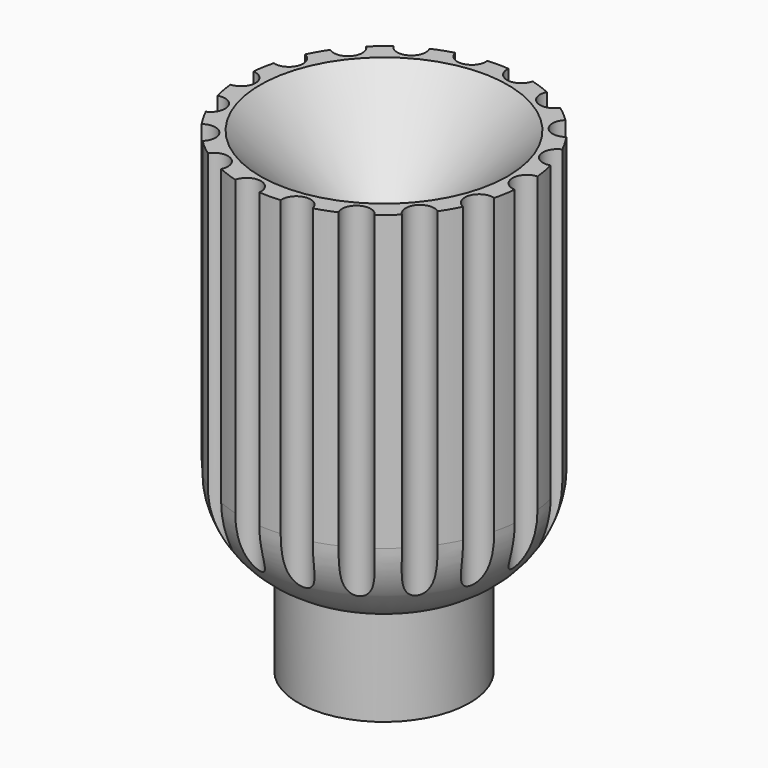
from build123d import *

# Parameters (mm, degrees)
F0_R     = 4.5
F0_R_2   = 1.5
F1_DEPTH = 5
F2_R     = 7.5
F2_R_2   = 1.5
F3_DEPTH = 20
F5_SIZE  = 5
F7_DEPTH = 25


# Not quite as in the source:
# - a fillet or chamfer that OpenCascade refuses, or shapes differently, is made with other operations: its cross-section is extruded or revolved along the edge and cut away or added


with BuildPart() as f1:
    # F0 (on Top) → F1 (new body)
    with BuildSketch(Plane.XY):
        Circle(F0_R)
        Circle(F0_R_2, mode=Mode.SUBTRACT)
    extrude(amount=F1_DEPTH)

    # F2 (on face) → F3 (join)
    with BuildSketch(Plane.XY.offset(5)):
        Circle(F2_R)
        Circle(F2_R_2, mode=Mode.SUBTRACT)
    extrude(amount=F3_DEPTH)

    # F4: fillet of radius 5 on 1 edges, made by hand

    # F4_s1 → F4_t2 (revolve, cut)
    with BuildSketch(Plane.XZ):
        with BuildLine():
            ThreePointArc((4.5, 5), (6.6833001327, 6.8439629074), (7.5, 9.582575695))
            Line((7.5, 9.582575695), (7.5, 5))
            Line((7.5, 5), (4.5, 5))
        make_face()
    revolve(axis=Axis((0, 0, 5), (0, 0, 1)), mode=Mode.SUBTRACT)

    # F5
    f5_edges = [f1.edges().sort_by_distance(p)[0] for p in [
        (-1.5, 0, 25),
    ]]
    chamfer(f5_edges, length=F5_SIZE)

    # F6 (on face) → F7 (cut)
    with BuildSketch(Plane.XY.offset(25)):
        with BuildLine():
            ThreePointArc((-7.4625, -0.7490619133), (-6.956573372, -0.5169018282), (-6.75, 0))
            ThreePointArc((-6.75, 0), (-6.956573372, 0.5169018282), (-7.4625, 0.7490619133))
            ThreePointArc((-7.4625, 0.7490619133), (-7.5, 0), (-7.4625, -0.7490619133))
        make_face()
        with BuildLine():
            ThreePointArc((-7.4625, -0.7490619133), (-7.5, 0), (-7.4625, 0.7490619133))
            ThreePointArc((-7.4625, 0.7490619133), (-8.25, 0), (-7.4625, -0.7490619133))
        make_face()
        with BuildLine():
            ThreePointArc((-6.7562619197, 3.256213272), (-7.0476946559, 2.5651510749), (-7.2686504456, 1.8484373671))
            ThreePointArc((-7.2686504456, 1.8484373671), (-6.60228296, 1.9617371033), (-6.2976946559, 2.5651510749))
            ThreePointArc((-6.2976946559, 2.5651510749), (-6.422764839, 2.9798349593), (-6.7562619197, 3.256213272))
        make_face()
        with BuildLine():
            ThreePointArc((-6.7562619197, -3.256213272), (-7.0476946559, -2.5651510749), (-7.2686504456, -1.8484373671))
            ThreePointArc((-7.2686504456, -1.8484373671), (-7.7524641215, -2.8216661824), (-6.7562619197, -3.256213272))
        make_face()
        with BuildLine():
            ThreePointArc((-6.2976946559, -2.5651510749), (-6.60228296, -1.9617371033), (-7.2686504456, -1.8484373671))
            ThreePointArc((-7.2686504456, -1.8484373671), (-7.0476946559, -2.5651510749), (-6.7562619197, -3.256213272))
            ThreePointArc((-6.7562619197, -3.256213272), (-6.422764839, -2.9798349593), (-6.2976946559, -2.5651510749))
        make_face()
        with BuildLine():
            ThreePointArc((-5.23511894, 5.3706172535), (-5.7453333234, 4.8209070726), (-6.1980943736, 4.222987821))
            ThreePointArc((-6.1980943736, 4.222987821), (-5.4114701685, 4.1493153858), (-4.9953333234, 4.8209070726))
            ThreePointArc((-4.9953333234, 4.8209070726), (-5.0578884938, 5.1207730531), (-5.23511894, 5.3706172535))
        make_face()
        with BuildLine():
            ThreePointArc((-4.9953333234, -4.8209070726), (-5.4114701685, -4.1493153858), (-6.1980943736, -4.222987821))
            ThreePointArc((-6.1980943736, -4.222987821), (-5.7453333234, -4.8209070726), (-5.23511894, -5.3706172535))
            ThreePointArc((-5.23511894, -5.3706172535), (-5.0578884938, -5.1207730531), (-4.9953333234, -4.8209070726))
        make_face()
        with BuildLine():
            ThreePointArc((-3.082543354, 6.8372455324), (-3.75, 6.4951905284), (-4.379956646, 6.0881836191))
            ThreePointArc((-4.379956646, 6.0881836191), (-3.5378296492, 5.7758270999), (-3, 6.4951905284))
            ThreePointArc((-3, 6.4951905284), (-3.020927821, 6.6711273289), (-3.082543354, 6.8372455324))
        make_face()
        with BuildLine():
            ThreePointArc((-3, -6.4951905284), (-3.5378296492, -5.7758270999), (-4.379956646, -6.0881836191))
            ThreePointArc((-4.379956646, -6.0881836191), (-3.75, -6.4951905284), (-3.082543354, -6.8372455324))
            ThreePointArc((-3.082543354, -6.8372455324), (-3.020927821, -6.6711273289), (-3, -6.4951905284))
        make_face()
        with BuildLine():
            ThreePointArc((-0.5581675461, 7.4792010931), (-1.3023613325, 7.3860581476), (-2.0335315056, 7.2190546206))
            ThreePointArc((-2.0335315056, 7.2190546206), (-1.2183304745, 6.6407804712), (-0.5523613325, 7.3860581476))
            ThreePointArc((-0.5523613325, 7.3860581476), (-0.5538142933, 7.4327200175), (-0.5581675461, 7.4792010931))
        make_face()
        with BuildLine():
            ThreePointArc((-0.5581675461, 7.4792010931), (-1.4325974658, 8.1246639624), (-2.0335315056, 7.2190546206))
            ThreePointArc((-2.0335315056, 7.2190546206), (-1.3023613325, 7.3860581476), (-0.5581675461, 7.4792010931))
        make_face()
        with BuildLine():
            ThreePointArc((-0.5523613325, -7.3860581476), (-1.2183304745, -6.6407804712), (-2.0335315056, -7.2190546206))
            ThreePointArc((-2.0335315056, -7.2190546206), (-1.3023613325, -7.3860581476), (-0.5581675461, -7.4792010931))
            ThreePointArc((-0.5581675461, -7.4792010931), (-0.5538142933, -7.4327200175), (-0.5523613325, -7.3860581476))
        make_face()
        with BuildLine():
            ThreePointArc((2.0335315056, 7.2190546206), (1.3023613325, 7.3860581476), (0.5581675461, 7.4792010931))
            ThreePointArc((0.5581675461, 7.4792010931), (1.1721251993, 6.6474523328), (2.0335315056, 7.2190546206))
        make_face()
        with BuildLine():
            ThreePointArc((2.0523613325, 7.3860581476), (1.3490232024, 8.1346051868), (0.5581675461, 7.4792010931))
            ThreePointArc((0.5581675461, 7.4792010931), (1.3023613325, 7.3860581476), (2.0335315056, 7.2190546206))
            ThreePointArc((2.0335315056, 7.2190546206), (2.0476390089, 7.3020272896), (2.0523613325, 7.3860581476))
        make_face()
        with BuildLine():
            ThreePointArc((2.0335315056, -7.2190546206), (1.1721251993, -6.6474523328), (0.5581675461, -7.4792010931))
            ThreePointArc((0.5581675461, -7.4792010931), (1.3023613325, -7.3860581476), (2.0335315056, -7.2190546206))
        make_face()
        with BuildLine():
            ThreePointArc((4.379956646, 6.0881836191), (3.75, 6.4951905284), (3.082543354, 6.8372455324))
            ThreePointArc((3.082543354, 6.8372455324), (3.375, 5.8456714755), (4.379956646, 6.0881836191))
        make_face()
        with BuildLine():
            ThreePointArc((4.5, 6.4951905284), (3.9259368005, 7.2242627074), (3.082543354, 6.8372455324))
            ThreePointArc((3.082543354, 6.8372455324), (3.75, 6.4951905284), (4.379956646, 6.0881836191))
            ThreePointArc((4.379956646, 6.0881836191), (4.4693634285, 6.2830201776), (4.5, 6.4951905284))
        make_face()
        with BuildLine():
            ThreePointArc((4.379956646, -6.0881836191), (3.375, -5.8456714755), (3.082543354, -6.8372455324))
            ThreePointArc((3.082543354, -6.8372455324), (3.75, -6.4951905284), (4.379956646, -6.0881836191))
        make_face()
        with BuildLine():
            ThreePointArc((6.1980943736, 4.222987821), (5.7453333234, 4.8209070726), (5.23511894, 5.3706172535))
            ThreePointArc((5.23511894, 5.3706172535), (5.1707999911, 4.3388163654), (6.1980943736, 4.222987821))
        make_face()
        with BuildLine():
            ThreePointArc((6.4953333234, 4.8209070726), (6.0451993038, 5.5083519023), (5.23511894, 5.3706172535))
            ThreePointArc((5.23511894, 5.3706172535), (5.7453333234, 4.8209070726), (6.1980943736, 4.222987821))
            ThreePointArc((6.1980943736, 4.222987821), (6.4169250102, 4.4870439178), (6.4953333234, 4.8209070726))
        make_face()
        with BuildLine():
            ThreePointArc((6.1980943736, -4.222987821), (5.1707999911, -4.3388163654), (5.23511894, -5.3706172535))
            ThreePointArc((5.23511894, -5.3706172535), (5.7453333234, -4.8209070726), (6.1980943736, -4.222987821))
        make_face()
        with BuildLine():
            ThreePointArc((7.2686504456, 1.8484373671), (7.0476946559, 2.5651510749), (6.7562619197, 3.256213272))
            ThreePointArc((6.7562619197, 3.256213272), (6.3429251903, 2.3086359674), (7.2686504456, 1.8484373671))
        make_face()
        with BuildLine():
            ThreePointArc((7.2686504456, -1.8484373671), (6.3429251903, -2.3086359674), (6.7562619197, -3.256213272))
            ThreePointArc((6.7562619197, -3.256213272), (7.0476946559, -2.5651510749), (7.2686504456, -1.8484373671))
        make_face()
        with BuildLine():
            ThreePointArc((7.5, 0), (7.4906191333, 0.375), (7.4625, 0.7490619133))
            ThreePointArc((7.4625, 0.7490619133), (6.75, 0), (7.4625, -0.7490619133))
            ThreePointArc((7.4625, -0.7490619133), (7.4906191333, -0.375), (7.5, 0))
        make_face()
        with BuildLine():
            ThreePointArc((8.25, 0), (8.0169018282, 0.543426628), (7.4625, 0.7490619133))
            ThreePointArc((7.4625, 0.7490619133), (7.4906191333, 0.375), (7.5, 0))
            ThreePointArc((7.5, 0), (7.4906191333, -0.375), (7.4625, -0.7490619133))
            ThreePointArc((7.4625, -0.7490619133), (8.0169018282, -0.543426628), (8.25, 0))
        make_face()
    extrude(amount=-F7_DEPTH, mode=Mode.SUBTRACT)


solid = f1.part
